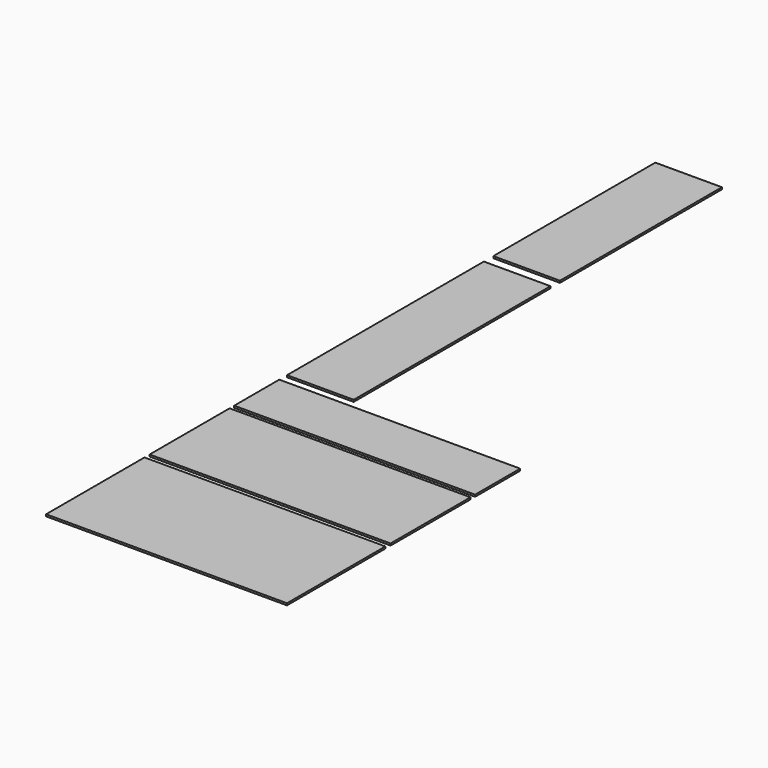
from build123d import *

# Parameters (mm, degrees)
F0_W     = 2387.6
F0_H     = 1219.2
F1_DEPTH = 19.05
F0_H_2   = 558.8
F0_W_2   = 660.4
F0_H_3   = 2438.4
F0_H_4   = 2006.6
F0_H_5   = 990.6


# Not quite as in the source:
# - a length typed as a fraction of an inch, garbled in the dataset ("3 / 203.2 mm" for 3/8 in), is restored


with BuildPart() as f1:
    # F0 (on Top) → F1 (new body)
    with BuildSketch(Plane.XY):
        with Locations((1193.8, 609.6)):
            Rectangle(F0_W, F0_H)
    extrude(amount=F1_DEPTH)


with BuildPart() as f1b:
    # F0 (on Top) → F1, piece 2 (new body)
    with BuildSketch(Plane.XY):
        with Locations((1193.8, 2609.6640914917)):
            Rectangle(F0_W, F0_H_2)
    extrude(amount=F1_DEPTH)


with BuildPart() as f1c:
    # F0 (on Top) → F1, piece 3 (new body)
    with BuildSketch(Plane.XY):
        with Locations((330.2, 4204.293832016)):
            Rectangle(F0_W_2, F0_H_3)
    extrude(amount=F1_DEPTH)


with BuildPart() as f1d:
    # F0 (on Top) → F1, piece 4 (new body)
    with BuildSketch(Plane.XY):
        with Locations((330.2, 6543.9432151794)):
            Rectangle(F0_W_2, F0_H_4)
    extrude(amount=F1_DEPTH)


with BuildPart() as f1e:
    # F0 (on Top) → F1, piece 5 (new body)
    with BuildSketch(Plane.XY):
        with Locations((1193.8, 1778.2109430313)):
            Rectangle(F0_W, F0_H_5)
    extrude(amount=F1_DEPTH)


solid = Compound([f1.part, f1b.part, f1c.part, f1d.part, f1e.part])
